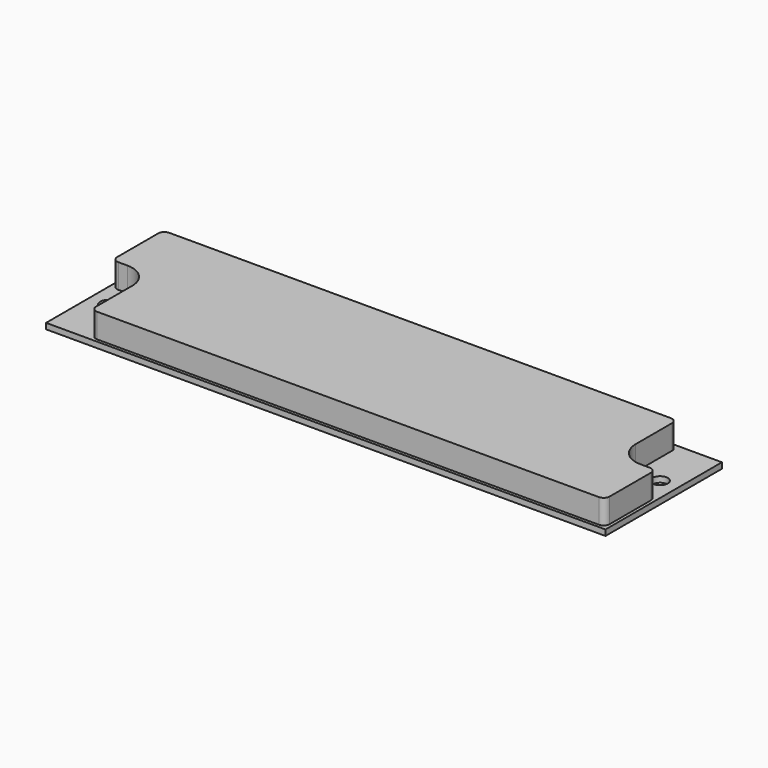
from build123d import *

# Parameters (mm, degrees)
F0_R     = 2
F0_R_2   = 4.7625
F1_DEPTH = 1.5
F3_DEPTH = 6.35


# Not quite as in the source:
# - a feature names something its author has since deleted; it is built from what else it names


with BuildPart() as f1:
    # F0 (on Top) → F1 (new body)
    with BuildSketch(Plane.XY):
        with BuildLine():
            Line((-73.025, 19), (-73.025, 1.5875))
            Line((-73.025, 1.5875), (-68.2625, 1.5875))
            ThreePointArc((-68.2625, 1.5875), (-61.9125, -4.7625), (-68.2625, -11.1125))
            Line((-68.2625, -11.1125), (-73.025, -11.1125))
            Line((-73.025, -11.1125), (-73.025, -19))
            Line((-73.025, -19), (73.025, -19))
            Line((73.025, -19), (73.025, -1.5875))
            Line((73.025, -1.5875), (68.2625, -1.5875))
            ThreePointArc((68.2625, -1.5875), (61.9125, 4.7625), (68.2625, 11.1125))
            Line((68.2625, 11.1125), (73.025, 11.1125))
            Line((73.025, 11.1125), (73.025, 19))
            Line((73.025, 19), (-73.025, 19))
        make_face()
        with BuildLine():
            Line((-73.025, 1.5875), (-73.025, -4.7625))
            Line((-73.025, -4.7625), (-73.025, -11.1125))
            Line((-73.025, -11.1125), (-68.2625, -11.1125))
            ThreePointArc((-68.2625, -11.1125), (-61.9125, -4.7625), (-68.2625, 1.5875))
            Line((-68.2625, 1.5875), (-73.025, 1.5875))
        make_face()
        with BuildLine():
            ThreePointArc((-73.025, -4.7625), (-68.2625, 0), (-63.5, -4.7625))
            ThreePointArc((-63.5, -4.7625), (-68.2625, -9.525), (-73.025, -4.7625))
        make_face(mode=Mode.SUBTRACT)
        with BuildLine():
            ThreePointArc((-73.025, -4.7625), (-68.2625, -9.525), (-63.5, -4.7625))
            ThreePointArc((-63.5, -4.7625), (-68.2625, 0), (-73.025, -4.7625))
        make_face()
        with Locations((-68.2625, -4.7625)):
            Circle(F0_R, mode=Mode.SUBTRACT)
        with BuildLine():
            Line((73.025, 4.7625), (73.025, 11.1125))
            Line((73.025, 11.1125), (68.2625, 11.1125))
            ThreePointArc((68.2625, 11.1125), (61.9125, 4.7625), (68.2625, -1.5875))
            Line((68.2625, -1.5875), (73.025, -1.5875))
            Line((73.025, -1.5875), (73.025, 4.7625))
        make_face()
        with Locations((68.2625, 4.7625)):
            Circle(F0_R_2, mode=Mode.SUBTRACT)
        with Locations((68.2625, 4.7625)):
            Circle(F0_R_2)
        with Locations((68.2625, 4.7625)):
            Circle(F0_R, mode=Mode.SUBTRACT)
    extrude(amount=F1_DEPTH)


with BuildPart() as f3:
    # F2 (on face) → F3 (new body)
    with BuildSketch(Plane.XY.offset(1.5)):
        with BuildLine():
            Line((70.637, -1.5875), (68.2625, -1.5875))
            ThreePointArc((68.2625, -1.5875), (63.7723719395, 0.2723719395), (61.9125, 4.7625))
            Line((61.9125, 4.7625), (61.9125, 16.612))
            ThreePointArc((61.9125, 16.612), (61.4473855685, 17.7348855685), (60.3245, 18.2))
            Line((60.3245, 18.2), (-70.637, 18.2))
            ThreePointArc((-70.637, 18.2), (-71.7598855685, 17.7348855685), (-72.225, 16.612))
            Line((-72.225, 16.612), (-72.225, 3.1755))
            ThreePointArc((-72.225, 3.1755), (-71.7598855685, 2.0526144315), (-70.637, 1.5875))
            Line((-70.637, 1.5875), (-68.2625, 1.5875))
            ThreePointArc((-68.2625, 1.5875), (-63.7723719395, -0.2723719395), (-61.9125, -4.7625))
            Line((-61.9125, -4.7625), (-61.9125, -16.612))
            ThreePointArc((-61.9125, -16.612), (-61.4473855685, -17.7348855685), (-60.3245, -18.2))
            Line((-60.3245, -18.2), (70.637, -18.2))
            ThreePointArc((70.637, -18.2), (71.7598855685, -17.7348855685), (72.225, -16.612))
            Line((72.225, -16.612), (72.225, -3.1755))
            ThreePointArc((72.225, -3.1755), (71.7598855685, -2.0526144315), (70.637, -1.5875))
        make_face()
    extrude(amount=F3_DEPTH)


solid = Compound([f1.part, f3.part])
